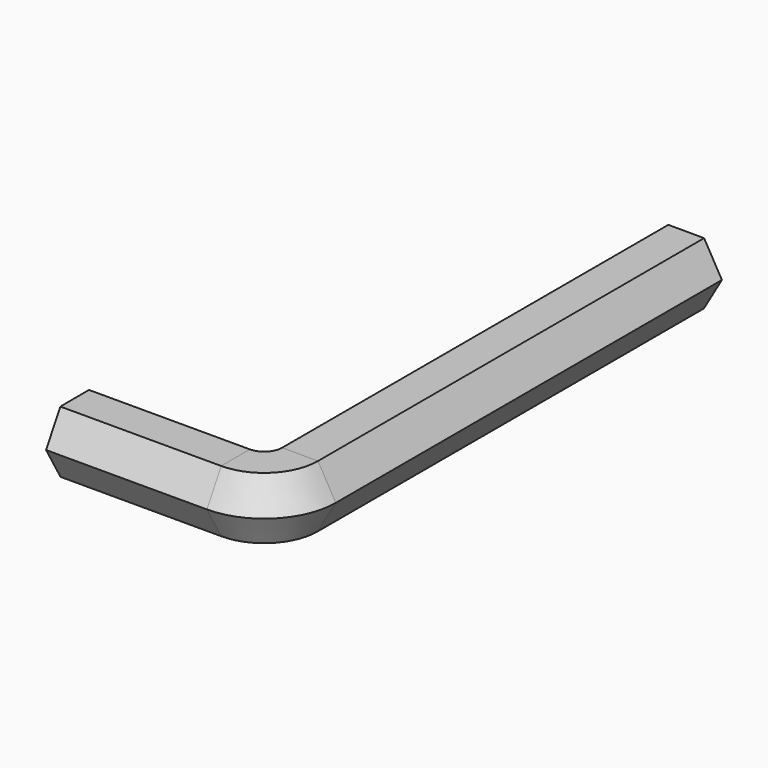
from build123d import *

# Parameters (mm, degrees)
F1_DEPTH = 150
F3_ANGLE = 90
F4_DEPTH = 50


with BuildPart() as f1:
    # F0 (on Front) → F1 (new body)
    with BuildSketch(Plane.XZ):
        Polygon((22.9738393507, -9.6457333625), (28.5607396108, -0.0310617447), (23.0276398708, 9.6146716177), (11.9076398708, 9.6457333625), (6.3207396108, 0.0310617447), (11.8538393507, -9.6146716177), align=None)
    extrude(amount=F1_DEPTH)

    # F2 (on face) → F3 (revolve)
    with BuildSketch(Plane.XZ.offset(150)):
        Polygon((11.9076398708, 9.6457333625), (6.3207396108, 0.0310617447), (11.8538393507, -9.6146716177), (22.9738393507, -9.6457333625), (28.5607396108, -0.0310617447), (23.0276398708, 9.6146716177), align=None)
    revolve(axis=Axis((6.3207396108, -150, 14.933847028), (0, 0, -1)), revolution_arc=F3_ANGLE)

    # F4 (add): a face of the model
    f4_faces = [f1.faces().sort_by_distance(p)[0] for p in [
        (6.3207396108, -161.12, 0),
    ]]
    extrude(f4_faces, amount=F4_DEPTH)


solid = f1.part
